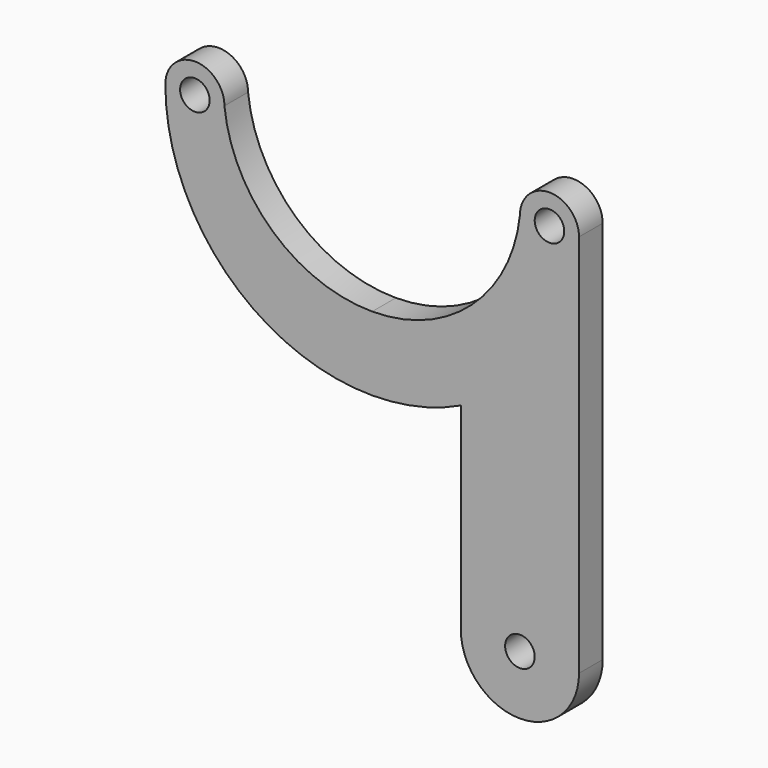
from build123d import *

# Parameters (mm, degrees)
F1_DEPTH = 6.35
F2_D     = 6.35


# Not quite as in the source:
# - a feature names something its author has since deleted; it is built from what else it names


with BuildPart() as f1:
    # F0 (on Front) → F1 (new body)
    with BuildSketch(Plane.XZ):
        with BuildLine():
            ThreePointArc((44.45, 0), (38.1, 6.35), (31.75, 0))
            ThreePointArc((31.75, 0), (38.1, -6.35), (44.45, 0))
        make_face()
        with BuildLine():
            Line((31.75, -31.1085197333), (31.75, 0))
            ThreePointArc((31.75, 0), (21.3576281747, -20.379309083), (0, -28.575))
            ThreePointArc((0, -28.575), (-21.3576281747, -20.379309083), (-31.75, 0))
            ThreePointArc((-31.75, 0), (-38.1, -6.35), (-44.45, 0))
            ThreePointArc((-44.45, 0), (-31.4308964237, -31.4308964237), (0, -44.45))
            ThreePointArc((0, -44.45), (9.7634350172, -43.3644766677), (19.05, -40.1609262841))
            ThreePointArc((19.05, -40.1609262841), (25.8001262805, -36.1960769132), (31.75, -31.1085197333))
        make_face()
        with BuildLine():
            ThreePointArc((44.45, 0), (38.1, -6.35), (31.75, 0))
            Line((31.75, 0), (31.75, -31.1085197333))
            ThreePointArc((31.75, -31.1085197333), (41.1527034349, -16.8005208253), (44.45, 0))
        make_face()
        with BuildLine():
            ThreePointArc((-44.45, 0), (-38.1, -6.35), (-31.75, 0))
            ThreePointArc((-31.75, 0), (-38.1, 6.35), (-44.45, 0))
        make_face()
        with BuildLine():
            Line((44.45, -44.45), (44.45, 0))
            ThreePointArc((44.45, 0), (41.1527034349, -16.8005208253), (31.75, -31.1085197333))
            Line((31.75, -31.1085197333), (31.75, -44.45))
            Line((31.75, -44.45), (44.45, -44.45))
        make_face()
        with BuildLine():
            Line((31.75, -44.45), (31.75, -31.1085197333))
            ThreePointArc((31.75, -31.1085197333), (25.8001262805, -36.1960769132), (19.05, -40.1609262841))
            Line((19.05, -40.1609262841), (19.05, -44.45))
            Line((19.05, -44.45), (31.75, -44.45))
        make_face()
        with BuildLine():
            Line((44.45, -82.55), (44.45, -44.45))
            Line((44.45, -44.45), (31.75, -44.45))
            Line((31.75, -44.45), (31.75, -69.85))
            ThreePointArc((31.75, -69.85), (40.7302561211, -73.5697438789), (44.45, -82.55))
        make_face()
        with BuildLine():
            Line((31.75, -69.85), (31.75, -44.45))
            Line((31.75, -44.45), (19.05, -44.45))
            Line((19.05, -44.45), (19.05, -82.55))
            ThreePointArc((19.05, -82.55), (22.7697438789, -73.5697438789), (31.75, -69.85))
        make_face()
        with BuildLine():
            Line((31.75, -82.55), (44.45, -82.55))
            ThreePointArc((44.45, -82.55), (40.7302561211, -73.5697438789), (31.75, -69.85))
            Line((31.75, -69.85), (31.75, -82.55))
        make_face()
        with BuildLine():
            ThreePointArc((19.05, -82.55), (31.75, -95.25), (44.45, -82.55))
            Line((44.45, -82.55), (31.75, -82.55))
            Line((31.75, -82.55), (19.05, -82.55))
        make_face()
        with BuildLine():
            Line((31.75, -82.55), (31.75, -69.85))
            ThreePointArc((31.75, -69.85), (22.7697438789, -73.5697438789), (19.05, -82.55))
            Line((19.05, -82.55), (31.75, -82.55))
        make_face()
    extrude(amount=F1_DEPTH)

    # F2 (through all)
    with Locations(Plane(origin=(0, 0, 0), x_dir=(1, 0, 0), z_dir=(0, 1, 0))):
        with Locations((-38.1, 0), (38.1, 0), (31.75, 82.55)):
            Hole(F2_D / 2)


solid = f1.part
